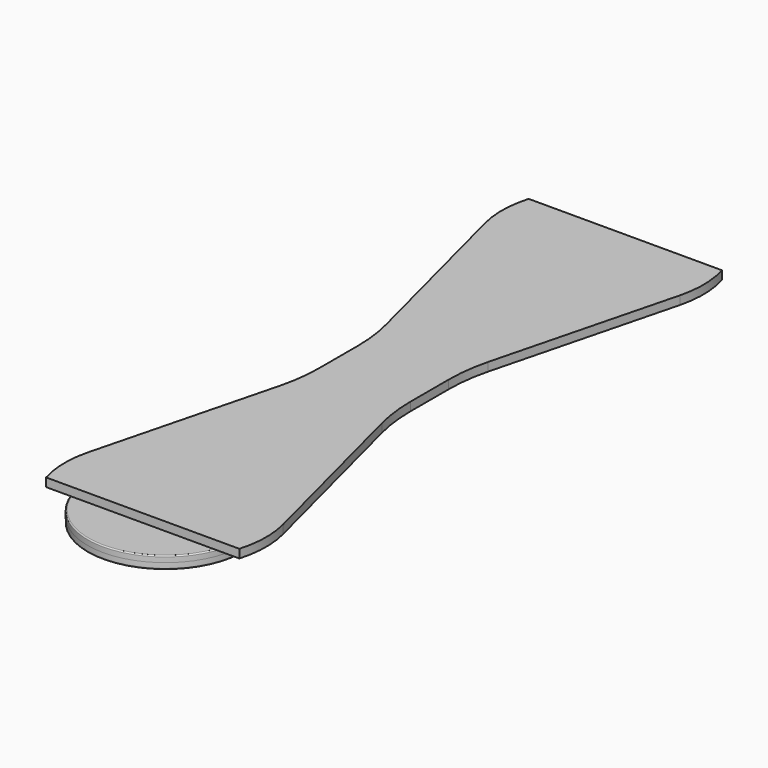
from build123d import *

# Parameters (mm, degrees)
F0_R         = 13.7
F1_DEPTH     = 1.075
F2_R         = 0.2
F3_TEXT_SIZE = 11.4102335532
F4_DEPTH     = 0.2
F6_COUNT     = 2
F6_ANGLE     = 180
F8_DEPTH     = 1.5


# Not quite as in the source:
# - Text() gives the source's letters only with a copy of the font that has no kerning and outlines rounded to 1/6400 em; it was checked with that copy


with BuildPart() as f1:
    # F0 (on Top) → F1 (new body)
    with BuildSketch(Plane.XY):
        Circle(F0_R)
    extrude(amount=F1_DEPTH)

    # F2
    f2_edges = [f1.edges().sort_by_distance(p)[0] for p in [
        (-13.7, 0, 1.075),
    ]]
    fillet(f2_edges, radius=F2_R)

    # F3 (on face) → F4 (join)
    with BuildSketch(Plane.XY.offset(1.075)):
        with Locations((-9.5, -4)):
            Text('2Fr.', F3_TEXT_SIZE, font='Open Sans', text_align=(TextAlign.LEFT, TextAlign.BOTTOM))
    extrude(amount=F4_DEPTH)

    # F6: F1 ×2 about axis
    f6_axis = Axis((0, 0, 0), (0, -1, 0))


with BuildPart() as f1_1:
    add(f1.part)
    for i in range(1, F6_COUNT):
        add(f1.part.rotate(f6_axis, i * F6_ANGLE / (F6_COUNT - 1)))


with BuildPart() as f8:
    # F7 (on Top) → F8 (new body)
    with BuildSketch(Plane.XY):
        with BuildLine():
            Line((0, 48), (6, 48))
            Line((6, 48), (6, 52.2085681882))
            ThreePointArc((6, 52.2085681882), (6.2525336206, 56.220846654), (7.0061486554, 60.1697979193))
            Line((7.0061486554, 60.1697979193), (15.2063583159, 92.0940216632))
            ThreePointArc((15.2063583159, 92.0940216632), (15.6896323919, 96.570469463), (14.8825401058, 101))
            Line((14.8825401058, 101), (-14.8825401058, 101))
            ThreePointArc((-14.8825401058, 101), (-15.6896323919, 96.570469463), (-15.2063583159, 92.0940216632))
            Line((-15.2063583159, 92.0940216632), (-7.0061486554, 60.1697979193))
            ThreePointArc((-7.0061486554, 60.1697979193), (-6.2525336206, 56.220846654), (-6, 52.2085681882))
            Line((-6, 52.2085681882), (-6, 48))
            Line((-6, 48), (0, 48))
        make_face()
        with BuildLine():
            Line((6, 52.2085681882), (6, 48))
            Line((6, 48), (8, 48))
            Line((8, 48), (8, 52.2085681882))
            ThreePointArc((8, 52.2085681882), (8.2367502693, 55.9700792499), (8.9432643645, 59.6722210611))
            Line((8.9432643645, 59.6722210611), (17.143474025, 91.596444805))
            ThreePointArc((17.143474025, 91.596444805), (17.6972966605, 96.309339476), (16.9791048056, 101))
            Line((16.9791048056, 101), (14.8825401058, 101))
            ThreePointArc((14.8825401058, 101), (15.6896323919, 96.570469463), (15.2063583159, 92.0940216632))
            Line((15.2063583159, 92.0940216632), (7.0061486554, 60.1697979193))
            ThreePointArc((7.0061486554, 60.1697979193), (6.2525336206, 56.220846654), (6, 52.2085681882))
        make_face()
        with BuildLine():
            Line((-8, 48), (-6, 48))
            Line((-6, 48), (-6, 52.2085681882))
            ThreePointArc((-6, 52.2085681882), (-6.2525336206, 56.220846654), (-7.0061486554, 60.1697979193))
            Line((-7.0061486554, 60.1697979193), (-15.2063583159, 92.0940216632))
            ThreePointArc((-15.2063583159, 92.0940216632), (-15.6896323919, 96.570469463), (-14.8825401058, 101))
            Line((-14.8825401058, 101), (-16.9791048056, 101))
            ThreePointArc((-16.9791048056, 101), (-17.6972966605, 96.309339476), (-17.143474025, 91.596444805))
            Line((-17.143474025, 91.596444805), (-8.9432643645, 59.6722210611))
            ThreePointArc((-8.9432643645, 59.6722210611), (-8.2367502693, 55.9700792499), (-8, 52.2085681882))
            Line((-8, 52.2085681882), (-8, 48))
        make_face()
        with BuildLine():
            Line((-14.8825401058, -5), (14.8825401058, -5))
            ThreePointArc((14.8825401058, -5), (15.6896323919, -0.570469463), (15.2063583159, 3.9059783368))
            Line((15.2063583159, 3.9059783368), (7.0061486554, 35.8302020807))
            ThreePointArc((7.0061486554, 35.8302020807), (6.2525336206, 39.779153346), (6, 43.7914318118))
            Line((6, 43.7914318118), (6, 48))
            Line((6, 48), (0, 48))
            Line((0, 48), (-6, 48))
            Line((-6, 48), (-6, 43.7914318118))
            ThreePointArc((-6, 43.7914318118), (-6.2525336206, 39.779153346), (-7.0061486554, 35.8302020807))
            Line((-7.0061486554, 35.8302020807), (-15.2063583159, 3.9059783368))
            ThreePointArc((-15.2063583159, 3.9059783368), (-15.6896323919, -0.570469463), (-14.8825401058, -5))
        make_face()
        with BuildLine():
            Line((-16.9791048056, -5), (-14.8825401058, -5))
            ThreePointArc((-14.8825401058, -5), (-15.6896323919, -0.570469463), (-15.2063583159, 3.9059783368))
            Line((-15.2063583159, 3.9059783368), (-7.0061486554, 35.8302020807))
            ThreePointArc((-7.0061486554, 35.8302020807), (-6.2525336206, 39.779153346), (-6, 43.7914318118))
            Line((-6, 43.7914318118), (-6, 48))
            Line((-6, 48), (-8, 48))
            Line((-8, 48), (-8, 43.7914318118))
            ThreePointArc((-8, 43.7914318118), (-8.2367502693, 40.0299207501), (-8.9432643645, 36.3277789389))
            Line((-8.9432643645, 36.3277789389), (-17.143474025, 4.403555195))
            ThreePointArc((-17.143474025, 4.403555195), (-17.6972966605, -0.309339476), (-16.9791048056, -5))
        make_face()
        with BuildLine():
            ThreePointArc((15.2063583159, 3.9059783368), (15.6896323919, -0.570469463), (14.8825401058, -5))
            Line((14.8825401058, -5), (16.9791048056, -5))
            ThreePointArc((16.9791048056, -5), (17.6972966605, -0.309339476), (17.143474025, 4.403555195))
            Line((17.143474025, 4.403555195), (8.9432643645, 36.3277789389))
            ThreePointArc((8.9432643645, 36.3277789389), (8.2367502693, 40.0299207501), (8, 43.7914318118))
            Line((8, 43.7914318118), (8, 48))
            Line((8, 48), (6, 48))
            Line((6, 48), (6, 43.7914318118))
            ThreePointArc((6, 43.7914318118), (6.2525336206, 39.779153346), (7.0061486554, 35.8302020807))
            Line((7.0061486554, 35.8302020807), (15.2063583159, 3.9059783368))
        make_face()
    extrude(amount=F8_DEPTH)


with BuildPart() as f8_1:
    # F9: moved
    add(f8.part.moved(Location((0, 0, 1.075))))


solid = Compound([f1_1.part, f8_1.part])
